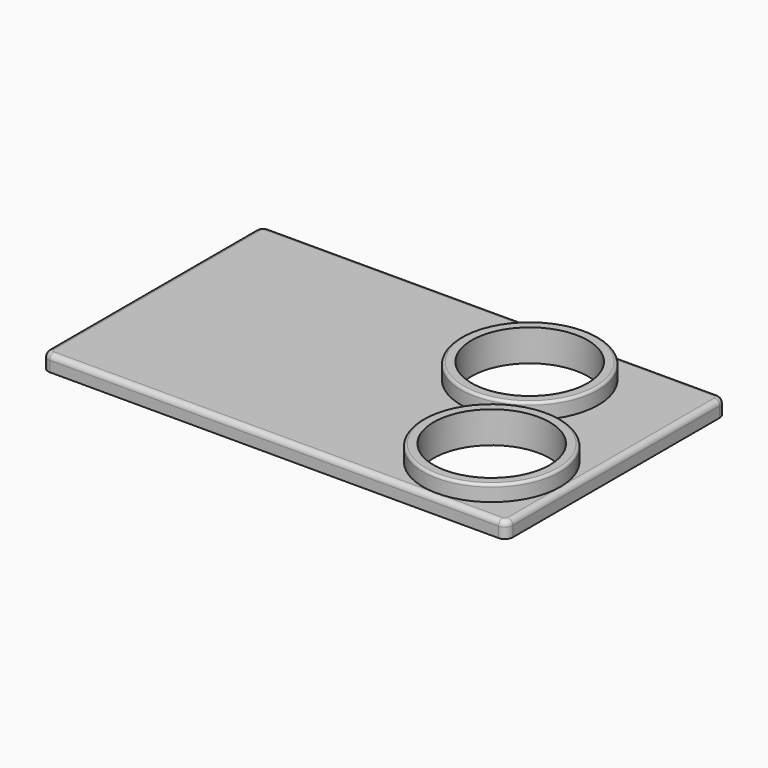
from build123d import *

# Parameters (mm, degrees)
F0_R         = 82.55
F0_R_2       = 69.85
F1_DEPTH     = 38.1
F0_W         = 558.8
F0_H         = 330.2
F2_DEPTH     = 19.05
F3_R         = 6.34999
F4_T1_DEPTH  = 42.8625
F4_T4_ANGLE  = 90
F4_T6_ANGLE  = 90
F4_T8_ANGLE  = 90
F4_T10_ANGLE = 90
F5_R         = 3.175


# Not quite as in the source:
# - a fillet or chamfer that OpenCascade refuses, or shapes differently, is made with other operations: its cross-section is extruded or revolved along the edge and cut away or added
# - a fillet or chamfer is up to 0.001 mm smaller than in the source, because OpenCascade refuses the exact size


with BuildPart() as f1:
    # F0 (on Top) → F1 (new body)
    with BuildSketch(Plane.XY):
        with Locations((393.7, 241.3)):
            Circle(F0_R)
        with Locations((393.7, 241.3)):
            Circle(F0_R_2, mode=Mode.SUBTRACT)
    extrude(amount=F1_DEPTH)



with BuildPart() as f1b:
    # F0 (on Top) → F1, piece 2 (new body)
    with BuildSketch(Plane.XY):
        with Locations((469.9, 88.9)):
            Circle(F0_R)
        with Locations((469.9, 88.9)):
            Circle(F0_R_2, mode=Mode.SUBTRACT)
    extrude(amount=F1_DEPTH)


with BuildPart() as f1_1:
    add(f1.part)

    add(f1b.part)  # F2 merges F1b
    # F0 (on Top) → F2 (join)
    with BuildSketch(Plane.XY):
        with Locations((279.4, 165.1)):
            Rectangle(F0_W, F0_H)
        with Locations((469.9, 88.9)):
            Circle(F0_R, mode=Mode.SUBTRACT)
        with Locations((393.7, 241.3)):
            Circle(F0_R, mode=Mode.SUBTRACT)
    extrude(amount=F2_DEPTH)

    # F3 (radius 6.35 in the source; OpenCascade refuses exactly that, so slightly less here)
    f3_edges = [f1_1.edges().sort_by_distance(p)[0] for p in [
        (0, 165.1, 19.05),
        (279.4, 330.2, 19.05),
        (279.4, 0, 19.05),
        (558.8, 165.1, 19.05),
    ]]
    fillet(f3_edges, radius=F3_R)

    # F4: fillet of radius 9.525 on 4 edges, made by hand

    # F4_s2 → F4_t1 (cut)
    with BuildSketch(Plane.XY.offset(-23.8125)):
        with BuildLine():
            ThreePointArc((0, 9.525), (2.7898079092, 2.7898079092), (9.525, 0))
            Line((9.525, 0), (0, 0))
            Line((0, 0), (0, 9.525))
        make_face()
        with BuildLine():
            ThreePointArc((549.275, 0), (556.0101920908, 2.7898079092), (558.8, 9.525))
            Line((558.8, 9.525), (558.8, 0))
            Line((558.8, 0), (549.275, 0))
        make_face()
        with BuildLine():
            ThreePointArc((549.275, 330.2), (556.0101920908, 327.4101920908), (558.8, 320.675))
            Line((558.8, 320.675), (558.8, 330.2))
            Line((558.8, 330.2), (549.275, 330.2))
        make_face()
        with BuildLine():
            ThreePointArc((0, 320.675), (2.7898079092, 327.4101920908), (9.525, 330.2))
            Line((9.525, 330.2), (0, 330.2))
            Line((0, 330.2), (0, 320.675))
        make_face()
    extrude(amount=F4_T1_DEPTH, mode=Mode.SUBTRACT)

    # F4_s3 → F4_t4 (revolve, cut)
    with BuildSketch(Plane.YZ.offset(9.525)):
        with BuildLine():
            ThreePointArc((323.85001, 19.05), (328.3401309895, 17.1901309895), (330.2, 12.70001))
            Line((330.2, 12.70001), (330.2, 19.05))
            Line((330.2, 19.05), (323.85001, 19.05))
        make_face()
    revolve(axis=Axis((9.525, 320.675, 19.05), (0, 0, 1)), revolution_arc=F4_T4_ANGLE, mode=Mode.SUBTRACT)

    # F4_s5 → F4_t6 (revolve, cut)
    with BuildSketch(Plane.XZ.offset(-320.675)):
        with BuildLine():
            ThreePointArc((552.45001, 19.05), (556.9401309895, 17.1901309895), (558.8, 12.70001))
            Line((558.8, 12.70001), (558.8, 19.05))
            Line((558.8, 19.05), (552.45001, 19.05))
        make_face()
    revolve(axis=Axis((549.275, 320.675, 19.05), (0, 0, 1)), revolution_arc=F4_T6_ANGLE, mode=Mode.SUBTRACT)

    # F4_s7 → F4_t8 (revolve, cut)
    with BuildSketch(Plane.YZ.offset(549.275)):
        with BuildLine():
            ThreePointArc((6.34999, 19.05), (1.8598690105, 17.1901309895), (0, 12.70001))
            Line((0, 12.70001), (0, 19.05))
            Line((0, 19.05), (6.34999, 19.05))
        make_face()
    revolve(axis=Axis((549.275, 9.525, 19.05), (0, 0, 1)), revolution_arc=F4_T8_ANGLE, mode=Mode.SUBTRACT)

    # F4_s9 → F4_t10 (revolve, cut)
    with BuildSketch(Plane.XZ.offset(-9.525)):
        with BuildLine():
            ThreePointArc((6.34999, 19.05), (1.8598690105, 17.1901309895), (0, 12.70001))
            Line((0, 12.70001), (0, 19.05))
            Line((0, 19.05), (6.34999, 19.05))
        make_face()
    revolve(axis=Axis((9.525, 9.525, 19.05), (0, 0, 1)), revolution_arc=F4_T10_ANGLE, mode=Mode.SUBTRACT)

    # F5
    f5_edges = [f1_1.edges().sort_by_distance(p)[0] for p in [
        (387.35, 88.9, 38.1),
        (311.15, 241.3, 38.1),
    ]]
    fillet(f5_edges, radius=F5_R)


solid = f1_1.part
